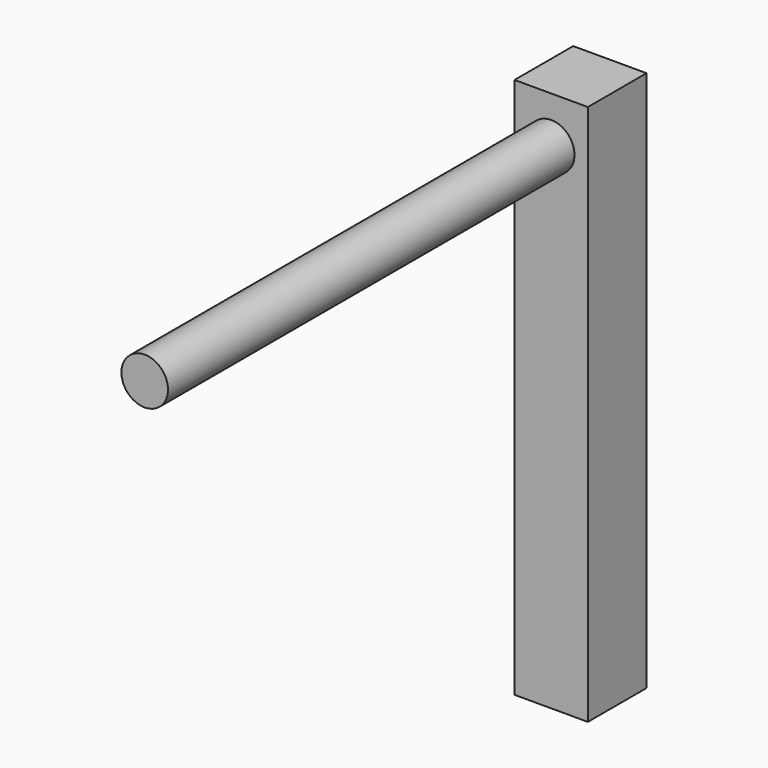
from build123d import *

# Parameters (mm, degrees)
F0_W     = 1.6002
F0_H     = 1.6002
F1_DEPTH = 11.811
F2_R     = 0.508
F3_DEPTH = 11.0871
F5_D     = 1.143
F5_DEPTH = 4.572
F5_TIP   = 0.3433918438


with BuildPart() as f1:
    # F0 (on Top) → F1 (new body)
    with BuildSketch(Plane.XY):
        Rectangle(F0_W, F0_H)
    extrude(amount=F1_DEPTH)

    # F2 (on face) → F3 (join)
    with BuildSketch(Plane.XZ.offset(0.8001)):
        with Locations((0, 10.795)):
            Circle(F2_R)
    extrude(amount=F3_DEPTH)

    # F5
    with Locations(Plane(origin=(0, 0, 0), x_dir=(1, 0, 0), z_dir=(0, 0, -1))):
        with Locations((0, 0)):
            Hole(F5_D / 2, depth=F5_DEPTH)
            with Locations((0, 0, -(F5_DEPTH + F5_TIP / 2))):  # 118° drill point
                Cone(0, F5_D / 2, F5_TIP, mode=Mode.SUBTRACT)


solid = f1.part
